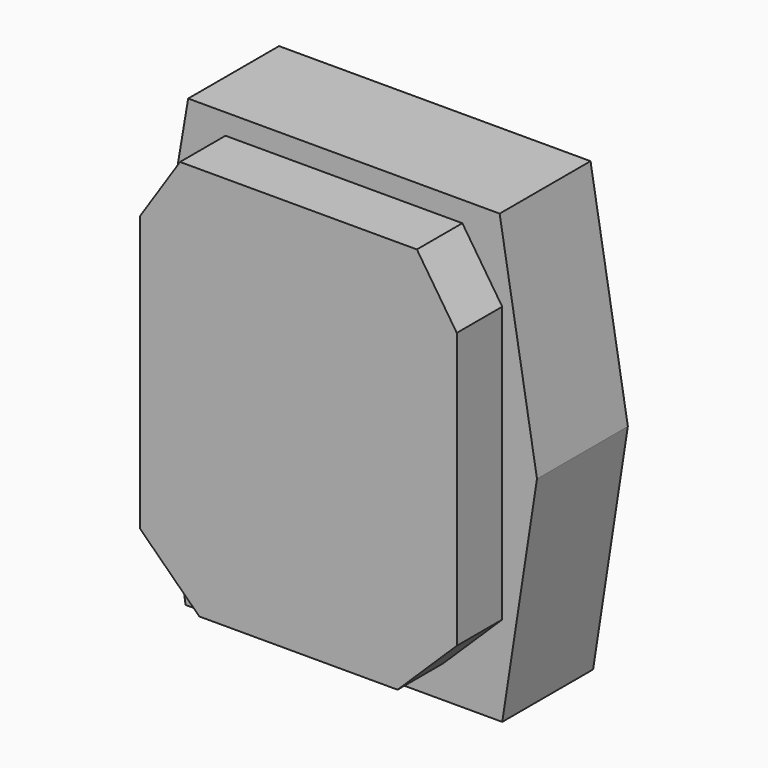
from build123d import *

# Parameters (mm, degrees)
F1_DEPTH = 25.4
F2_DEPTH = 12.7
F4_DEPTH = 25.4


# Not quite as in the source:
# - the program builds the solid bodies; features that only make, move or delete a surface that nothing else refers to are left out


with BuildPart() as f1:
    # F0 (on Front) → F1 (new body)
    with BuildSketch(Plane.XZ):
        Polygon((-22.1610441804, -43.1708656251), (0, -43.1708656251), (22.1610441804, -43.1708656251), (35.4001075029, -30.2196051925), (35.4001075029, 31.3708260655), (26.4781303704, 44.897697866), (0, 44.897697866), (-26.4781303704, 44.897697866), (-35.4001075029, 31.3708260655), (-35.4001075029, -30.2196051925), align=None)
    extrude(amount=F1_DEPTH)

    # F2 (cut): a face of the model
    f2_faces = [f1.faces().sort_by_distance(p)[0] for p in [
        (0, -25.4, 1.2066431814),
    ]]
    extrude(f2_faces, amount=-F2_DEPTH, mode=Mode.SUBTRACT)

    # F3 (on Front) → F4 (join)
    with BuildSketch(Plane.XZ):
        Polygon((34.8244979978, 49.5025888085), (0, 49.5025888085), (-34.8244979978, 49.5025888085), (-43.1708618999, 0), (-35.4001075029, -50.3660067916), (0, -50.3660067916), (35.4001075029, -50.3660067916), (43.1708618999, 0), align=None)
    extrude(amount=-F4_DEPTH)


solid = f1.part
